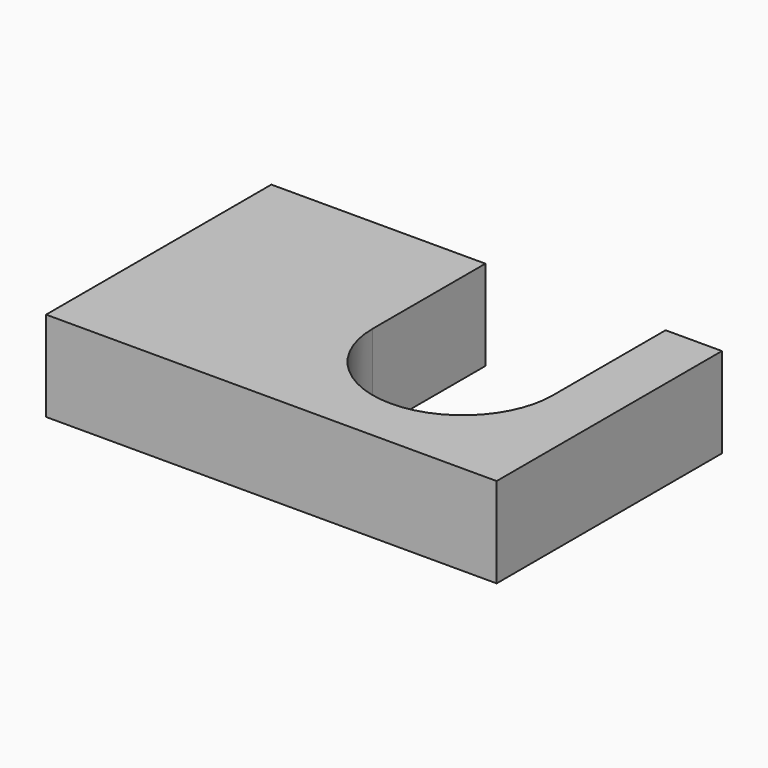
from build123d import *

# Parameters (mm, degrees)
F0_W     = 40
F0_H     = 25
F0_R     = 8
F1_DEPTH = 8
F3_DEPTH = 8


# Not quite as in the source:
# - a feature of the source that left no trace in its solid (it failed there, or was rolled back) is left out


with BuildPart() as f1:
    # F0 (on Top) → F1 (new body)
    with BuildSketch(Plane.XY):
        Rectangle(F0_W, F0_H)
        with Locations((7, 0)):
            Circle(F0_R, mode=Mode.SUBTRACT)
    extrude(amount=F1_DEPTH)

    # F2 (on face) → F3 (cut, through all)
    with BuildSketch(Plane.XY.offset(8)):
        with BuildLine():
            Line((-1, 12.5), (-1, 0))
            ThreePointArc((-1, 0), (7, 8), (15, 0))
            Line((15, 0), (15, 12.5))
            Line((15, 12.5), (-1, 12.5))
        make_face()
    extrude(amount=-F3_DEPTH, mode=Mode.SUBTRACT)


solid = f1.part
